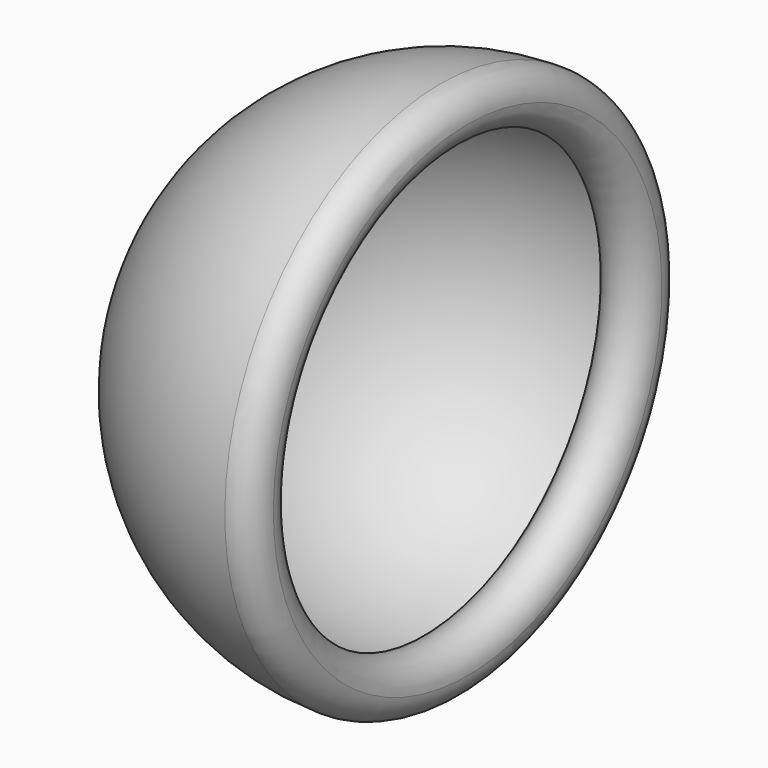
from build123d import *

# Parameters (mm, degrees)
F2_R        = 1.25
F3_DEPTH    = 20.848816548
F4_T2_ANGLE = 269.9999999999
F4_T4_ANGLE = 90.0000002223


# Not quite as in the source:
# - a fillet or chamfer that OpenCascade refuses, or shapes differently, is made with other operations: its cross-section is extruded or revolved along the edge and cut away or added


with BuildPart() as f1:
    # F0 (on Front) → F1 (revolve)
    with BuildSketch(Plane.XZ):
        with BuildLine():
            ThreePointArc((20.847816448, 19.2961636657), (20.2143632876, 20.8119613812), (18.6907213238, 21.4263072013))
            ThreePointArc((18.6907213238, 21.4263072013), (16.8507396209, 20.3225249849), (16.9045229372, 18.1775365926))
            ThreePointArc((16.9045229372, 18.1775365926), (19.2988876007, 17.2467192141), (20.847816448, 19.2961636657))
        make_face()
        with BuildLine():
            Line((-1.75, 5.5), (0, 5.5))
            Line((0, 5.5), (0, 0))
            Line((0, 0), (0.6667277431, 0))
            ThreePointArc((0.6667277431, 0), (5.3173187467, 12.1869687509), (16.9045229372, 18.1775365926))
            ThreePointArc((16.9045229372, 18.1775365926), (16.8507396209, 20.3225249849), (18.6907213238, 21.4263072013))
            ThreePointArc((18.6907213238, 21.4263072013), (5.7901979365, 16.9030256739), (-1.75, 5.5))
        make_face()
    revolve(axis=Axis((0.3358235447, 0, 0), (1, 0, 0)))

    # F2 (on face) → F3 (cut, through all)
    with BuildSketch(Plane(origin=(0, 0, 0), x_dir=(0, -1, 0), z_dir=(-1, 0, 0))):
        Circle(F2_R)
    extrude(amount=-F3_DEPTH, mode=Mode.SUBTRACT)

    # F4: chamfer of 0.5 on 2 edges, made by hand

    # F4_s1 → F4_t2 (revolve, cut)
    with BuildSketch(Plane.XZ):
        with BuildLine():
            Line((0.7639536686, 1.7481015134), (0.2013545471, 1.2365450652))
            Line((0.2013545471, 1.2365450652), (0.2013545471, 1.2265450652))
            ThreePointArc((0.2013545471, 1.2265450652), (0.4554194631, 1.24), (0.7094843791, 1.24))
            Line((0.7094843791, 1.24), (0.7194610064, 1.2493166933))
            ThreePointArc((0.7194610064, 1.2493166933), (0.7382742313, 1.4989228259), (0.7739086095, 1.7471532769))
            Line((0.7739086095, 1.7471532769), (0.7639536686, 1.7481015134))
        make_face()
    revolve(axis=Axis((0.7094843791, 0, 0), (-1, 0, 0)), revolution_arc=F4_T2_ANGLE, mode=Mode.SUBTRACT)

    # F4_s3 → F4_t4 (revolve, cut)
    with BuildSketch(Plane.XY.offset(2.5e-09)):
        with BuildLine():
            Line((0.7639536686, -1.7481015124), (0.2013545471, -1.2365450642))
            Line((0.2013545471, -1.2365450642), (0.2013545471, -1.2265450642))
            ThreePointArc((0.2013545471, -1.2265450642), (0.4554194631, -1.239999999), (0.7094843791, -1.24))
            Line((0.7094843791, -1.24), (0.7194610064, -1.2493166933))
            ThreePointArc((0.7194610064, -1.2493166933), (0.7382742313, -1.4989228254), (0.7739086095, -1.7471532759))
            Line((0.7739086095, -1.7471532759), (0.7639536686, -1.7481015124))
        make_face()
    revolve(axis=Axis((0.7094843791, -2.4e-09, 2.5e-09), (-1, 0, 0)), revolution_arc=F4_T4_ANGLE, mode=Mode.SUBTRACT)


solid = f1.part
